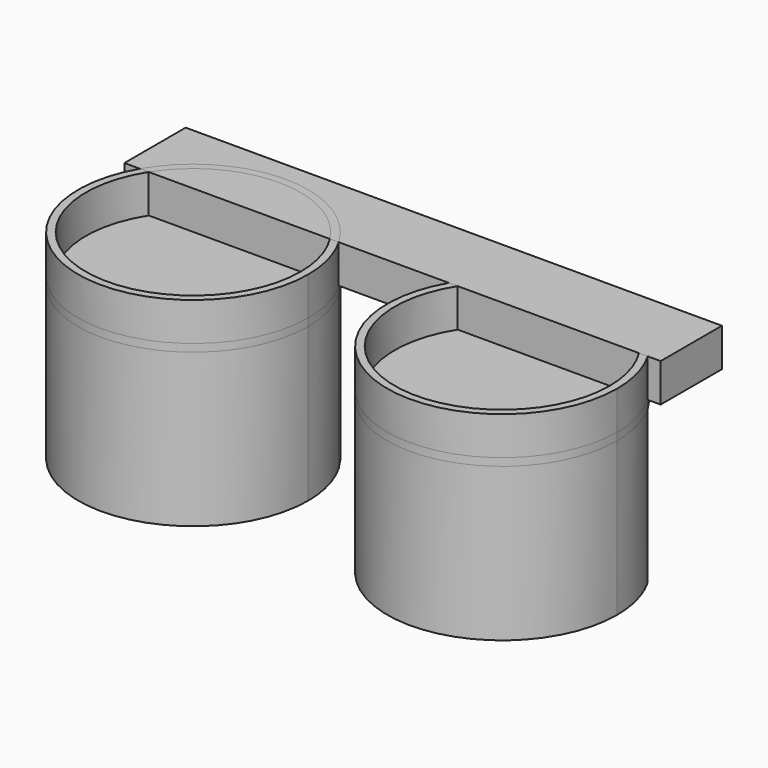
from build123d import *
from build123d import SkipClean  # not in build123d's __all__

# Parameters (mm, degrees)
F0_W     = 177.8
F0_H     = 12.7
F1_DEPTH = 25.4
F3_DEPTH = 66.04
F4_R     = 38.1
F5_DEPTH = 2.54


with BuildPart() as f1:
    # F0 (on Front) → F1 (new body)
    with BuildSketch(Plane.XZ):
        Rectangle(F0_W, F0_H)
    extrude(amount=F1_DEPTH)



with BuildPart() as f3:
    # F2 (on face) → F3 (new body)
    with BuildSketch(Plane.XY.offset(6.35)):
        with BuildLine():
            ThreePointArc((-83.7517897457, -25.4), (-60.6861906119, -81.3033672223), (-12.6913306355, -44.5106811821))
            ThreePointArc((-12.6913306355, -44.5106811821), (-13.9986445954, -34.6158212058), (-17.8308715254, -25.4))
            Line((-17.8308715254, -25.4), (-20.7487240634, -25.4))
            ThreePointArc((-20.7487240634, -25.4), (-16.6045729668, -34.558699219), (-15.1854835751, -44.5106811821))
            ThreePointArc((-15.1854835751, -44.5106811821), (-60.7433125987, -78.6974388509), (-80.8339372077, -25.4))
            Line((-80.8339372077, -25.4), (-83.7517897457, -25.4))
        make_face()
        with BuildLine():
            Line((-20.7487240634, -25.4), (-17.8308715254, -25.4))
            ThreePointArc((-17.8308715254, -25.4), (-50.7913306355, -6.4106811821), (-83.7517897457, -25.4))
            Line((-83.7517897457, -25.4), (-80.8339372077, -25.4))
            ThreePointArc((-80.8339372077, -25.4), (-50.7913306355, -8.9048341217), (-20.7487240634, -25.4))
        make_face()
    extrude(amount=-F3_DEPTH)


with BuildPart() as f3b:
    # F2 (on face) → F3, piece 2 (new body)
    with BuildSketch(Plane.XY.offset(6.35)):
        with BuildLine():
            Line((21.6144230301, -25.4), (18.7024404436, -25.4))
            ThreePointArc((18.7024404436, -25.4), (41.7680395775, -81.3033672223), (89.7628995538, -44.5106811821))
            ThreePointArc((89.7628995538, -44.5106811821), (88.4555855939, -34.6158212058), (84.623358664, -25.4))
            Line((84.623358664, -25.4), (81.7113760775, -25.4))
            ThreePointArc((81.7113760775, -25.4), (85.8548530255, -34.5588273636), (87.2736995538, -44.5106811821))
            ThreePointArc((87.2736995538, -44.5106811821), (41.7110457353, -78.7026346539), (21.6144230301, -25.4))
        make_face()
    extrude(amount=-F3_DEPTH)


with BuildPart() as f1_1:
    add(f1.part, clean=False)

    with SkipClean():  # cleaning this boolean's faces spoils the solid; the shape is the same uncleaned
        add(f3.part)  # F5 merges F3

    with SkipClean():  # cleaning this boolean's faces spoils the solid; the shape is the same uncleaned
        add(f3b.part)  # F5 merges F3b
    # F4 (on face) → F5 (join)
    with BuildSketch(Plane(origin=(0, 0, -6.35), x_dir=(1, 0, 0), z_dir=(0, 0, -1))):
        with Locations((-50.7913306355, 44.5106811821)):
            Circle(F4_R)
        with Locations((51.6628995538, 44.5106811821)):
            Circle(F4_R)
    with SkipClean():  # cleaning this boolean's faces spoils the solid; the shape is the same uncleaned
        extrude(amount=F5_DEPTH)


solid = f1_1.part
